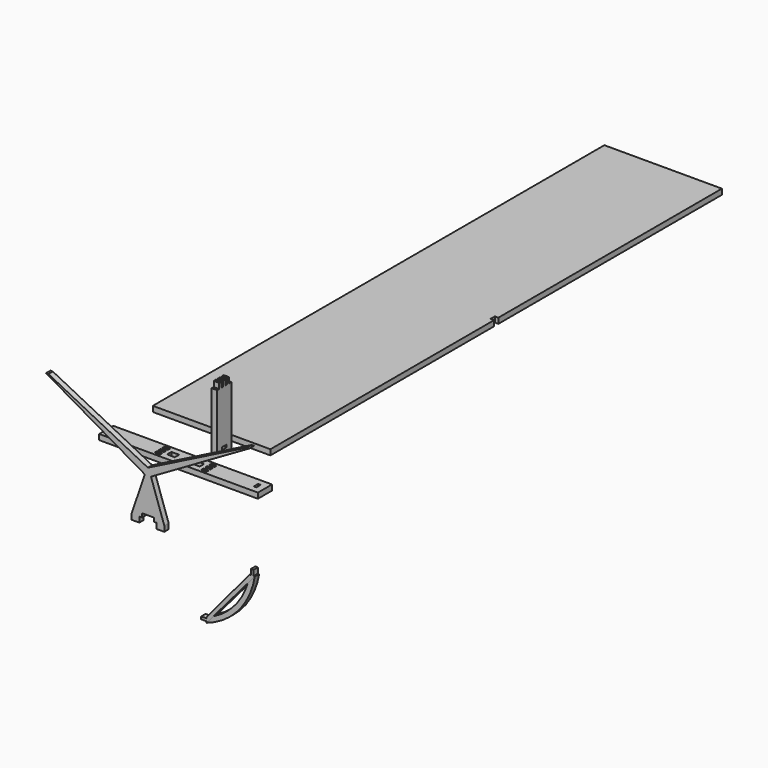
from build123d import *

# Parameters (mm, degrees)
F1_W      = 5.8928
F1_H      = 2.794
F1_W_2    = 2.794
F1_H_2    = 5.8928
F2_DEPTH  = 5.8928
F3_W      = 2.794
F3_H      = 12.9595901101
F3_W_2    = 2.54
F3_H_2    = 5.8928
F4_DEPTH  = 5.8928
F5_W      = 2.794
F5_H      = 5.8928
F5_W_2    = 5.8928
F5_H_2    = 2.794
F6_DEPTH  = 5.8928
F7_W      = 2.794
F7_H      = 5.8928
F7_W_2    = 5.8928
F7_H_2    = 2.794
F8_DEPTH  = 5.8928
F10_DEPTH = 5.8928
F13_DEPTH = 5.8928


# Not quite as in the source:
# - a variable given as a bare number and used for a length is read in inches; the dataset says mm whatever the document's units were


with BuildPart() as f2:
    # F1 (on Top) → F2 (new body)
    with BuildSketch(Plane.XY):
        Polygon((22.4183307789, 37.9304943726), (10.7343307789, 37.9304943726), (10.7343307789, 31.3518943726), (14.9253307789, 31.3518943726), (14.9253307789, 25.4590943726), (10.7343307789, 25.4590943726), (10.7343307789, 18.8804943726), (22.4183307789, 18.8804943726), (74.6153307789, 18.8804943726), (74.6153307789, 25.4590943726), (73.2183307789, 25.4590943726), (73.2183307789, 31.3518943726), (74.6153307789, 31.3518943726), (74.6153307789, 37.9304943726), align=None)
        Polygon((25.3647307789, 21.6744943726), (22.4183307789, 21.6744943726), (19.4719307789, 21.6744943726), (19.4719307789, 24.4684943726), (25.3647307789, 24.4684943726), align=None, mode=Mode.SUBTRACT)
        with Locations((22.4183307789, 28.4054943726)):
            Rectangle(F1_W, F1_H, mode=Mode.SUBTRACT)
        Polygon((19.4719307789, 35.1364943726), (22.4183307789, 35.1364943726), (25.3647307789, 35.1364943726), (25.3647307789, 32.3424943726), (19.4719307789, 32.3424943726), align=None, mode=Mode.SUBTRACT)
        Polygon((-2.7530692211, 37.9304943726), (-88.4780692211, 37.9304943726), (-88.4780692211, 18.8804943726), (-2.7530692211, 18.8804943726), (-2.7530692211, 28.4054943726), align=None)
        with Locations((-27.9244692211, 23.0714943726)):
            Rectangle(F1_W, F1_H, mode=Mode.SUBTRACT)
        with Locations((-80.1214692211, 28.4054943726)):
            Rectangle(F1_W_2, F1_H_2, mode=Mode.SUBTRACT)
        with Locations((-27.9244692211, 28.4054943726)):
            Rectangle(F1_W, F1_H, mode=Mode.SUBTRACT)
        Polygon((-12.0494692211, 31.3518943726), (-12.0494692211, 28.4054943726), (-12.0494692211, 25.4590943726), (-20.4314692211, 25.4590943726), (-20.4314692211, 31.3518943726), align=None, mode=Mode.SUBTRACT)
        with Locations((-27.9244692211, 33.7394943726)):
            Rectangle(F1_W, F1_H, mode=Mode.SUBTRACT)
        Polygon((82.9719307789, 37.9304943726), (74.6153307789, 37.9304943726), (74.6153307789, 31.3518943726), (76.0123307789, 31.3518943726), (76.0123307789, 25.4590943726), (74.6153307789, 25.4590943726), (74.6153307789, 18.8804943726), (82.9719307789, 18.8804943726), align=None)
        Polygon((10.7343307789, 37.9304943726), (-2.7530692211, 37.9304943726), (-2.7530692211, 28.4054943726), (6.5433307789, 28.4054943726), (6.5433307789, 31.3518943726), (10.7343307789, 31.3518943726), align=None)
        Polygon((6.5433307789, 28.4054943726), (-2.7530692211, 28.4054943726), (-2.7530692211, 18.8804943726), (10.7343307789, 18.8804943726), (10.7343307789, 25.4590943726), (6.5433307789, 25.4590943726), align=None)
    extrude(amount=F2_DEPTH)


with BuildPart() as f4:
    # F3 (on Right) → F4 (new body)
    with BuildSketch(Plane.YZ):
        Polygon((60.25341, -2.19075), (79.30341, -2.19075), (79.30341, 4.572), (72.72481, 4.572), (72.72481, 1.778), (66.83201, 1.778), (66.83201, 4.572), (60.25341, 4.572), align=None)
        Polygon((72.72481, 4.572), (79.30341, 4.572), (79.30341, 48.3496598899), (76.50941, 48.3496598899), (73.71541, 48.3496598899), (71.17541, 48.3496598899), (68.38141, 48.3496598899), (65.84141, 48.3496598899), (63.04741, 48.3496598899), (60.25341, 48.3496598899), (60.25341, 4.572), (66.83201, 4.572), align=None)
        Polygon((76.50941, 48.3496598899), (79.30341, 48.3496598899), (79.30341, 54.61), (79.30341, 61.30925), (76.50941, 61.30925), align=None)
        with Locations((61.65041, 54.829454945)):
            Rectangle(F3_W, F3_H)
        with Locations((75.11241, 54.829454945)):
            Rectangle(F3_W, F3_H)
        with Locations((64.44441, 54.829454945)):
            Rectangle(F3_W, F3_H)
        with Locations((72.44541, 54.829454945)):
            Rectangle(F3_W_2, F3_H)
        with Locations((75.11241, 64.25565)):
            Rectangle(F3_W, F3_H_2)
        with Locations((64.44441, 64.25565)):
            Rectangle(F3_W, F3_H_2)
        with Locations((67.11141, 54.829454945)):
            Rectangle(F3_W_2, F3_H)
        with Locations((69.77841, 54.829454945)):
            Rectangle(F3_W, F3_H)
        with Locations((69.77841, 64.25565)):
            Rectangle(F3_W, F3_H_2)
    extrude(amount=F4_DEPTH)


with BuildPart() as f6:
    # F5 (on Front) → F6 (new body)
    with BuildSketch(Plane.XZ):
        with BuildLine():
            Line((95.2629311906, -58.4977063152), (93.8659311906, -58.4977063152))
            ThreePointArc((93.8659311906, -58.4977063152), (78.2238370796, -92.5362400683), (47.4093311906, -113.8379563152))
            Line((47.4093311906, -113.8379563152), (47.4093311906, -115.2349563152))
            Line((47.4093311906, -115.2349563152), (47.4093311906, -118.0289563152))
            Line((47.4093311906, -118.0289563152), (47.4093311906, -119.4259563152))
            ThreePointArc((47.4093311906, -119.4259563152), (81.937577657, -96.2275673485), (99.4539311906, -58.4977063152))
            Line((99.4539311906, -58.4977063152), (98.0569311906, -58.4977063152))
            Line((98.0569311906, -58.4977063152), (95.2629311906, -58.4977063152))
        make_face()
        with Locations((96.6599311906, -55.5513063152)):
            Rectangle(F5_W, F5_H)
        with Locations((44.4629311906, -116.6319563152)):
            Rectangle(F5_W_2, F5_H_2)
    extrude(amount=F6_DEPTH)


with BuildPart() as f8:
    # F7 (on Front) → F8 (new body)
    with BuildSketch(Plane.XZ):
        Polygon((98.0569311906, -58.4977063152), (95.2629311906, -58.4977063152), (93.8659311906, -58.4977063152), (47.4093311906, -113.8379563152), (47.4093311906, -115.2349563152), (47.4093311906, -118.0289563152), (47.4093311906, -119.4259563152), (99.4539311906, -58.4977063152), align=None)
        with Locations((96.6599311906, -55.5513063152)):
            Rectangle(F7_W, F7_H)
        with Locations((44.4629311906, -116.6319563152)):
            Rectangle(F7_W_2, F7_H_2)
    extrude(amount=F8_DEPTH)


with BuildPart() as f10:
    # F9 (on Front) → F10 (new body)
    with BuildSketch(Plane.XZ):
        Polygon((-123.4517790751, 61.595), (-125.9917790751, 61.595), (-19.3061095829, 0), (-16.0065527945, 0), (-16.0065527945, 7.4160954057), align=None)
        Polygon((-16.0065527945, -1.905), (-19.3061095829, 0), (-33.6849527945, -41.9280635703), (-33.6849527945, -47.8208635703), (-25.3029527945, -47.8208635703), (-25.3029527945, -41.9280635703), (-22.3565527945, -41.9280635703), (-22.3565527945, -37.8640635703), (-16.0065527945, -37.8640635703), align=None)
        Polygon((-16.0065527945, 0), (-19.3061095829, 0), (-16.0065527945, -1.905), align=None)
        Polygon((91.4386734861, 61.595), (-16.0065527945, 7.4160954057), (-16.0065527945, 0), (-12.7069960061, 0), (93.9786734861, 61.595), align=None)
        Polygon((-12.7069960061, 0), (-16.0065527945, 0), (-16.0065527945, -1.905), align=None)
        Polygon((-12.7069960061, 0), (-16.0065527945, -1.905), (-16.0065527945, -37.8640635703), (-9.6565527945, -37.8640635703), (-9.6565527945, -41.9280635703), (-6.7101527945, -41.9280635703), (-6.7101527945, -47.8208635703), (1.6718472055, -47.8208635703), (1.6718472055, -41.9280635703), align=None)
    extrude(amount=F10_DEPTH)


with BuildPart() as f13:
    # F12 (on Top) → F13 (new body)
    with BuildSketch(Plane.XY):
        Polygon((41.7525291319, 696.9023720026), (-85.2474708681, 696.9023720026), (-85.2474708681, 87.3023720026), (41.7525291319, 87.3023720026), (41.7525291319, 389.1559720026), (37.9425291319, 389.1559720026), (37.9425291319, 395.0487720026), (41.7525291319, 395.0487720026), align=None)
    extrude(amount=F13_DEPTH)


solid = Compound([f2.part, f4.part, f6.part, f8.part, f10.part, f13.part])
